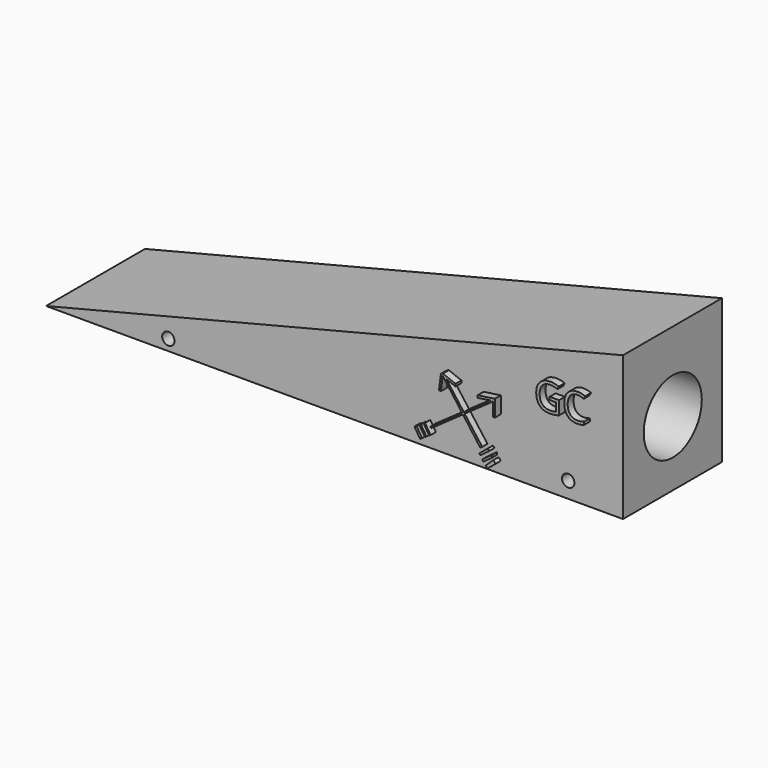
from build123d import *

# Parameters (mm, degrees)
F1_DEPTH     = 38.1
F4_DEPTH     = 2.032
F5_DEPTH     = 2.286
F6_R         = 11.180279411
F7_DEPTH     = 50.8
F8_TEXT_SIZE = 11.8700451114
F9_DEPTH     = 2.286
F11_DEPTH    = 3.302
F13_DEPTH    = 2.54
F14_R        = 1.905
F15_R        = 1.905
F16_DEPTH    = 58.166


# Not quite as in the source:
# - Text() gives the source's letters only with a copy of the font that has no kerning and outlines rounded to 1/6400 em; it was checked with that copy


with BuildPart() as f1:
    # F0 (on Front) → F1 (new body)
    with BuildSketch(Plane.XZ):
        Polygon((84.4861016917, 44.45), (-93.3138983083, 0), (84.4861016917, 0), align=None)
    extrude(amount=F1_DEPTH)

    # F2 (on face) → F4 (join)
    with BuildSketch(Plane.XZ.offset(38.1)):
        Polygon((36.5162249075, 14.0483667249), (26.7250510784, 7.1465180973), (26.9805269975, 6.7933419292), (36.7746398831, 13.6972623128), align=None)
        Polygon((30.2000753582, 22.6300209761), (36.5162249075, 14.0483667249), (37.0527973612, 14.4265993982), (30.6655891783, 22.9777331921), align=None)
        Polygon((37.0527973612, 14.4265993982), (36.5162249075, 14.0483667249), (36.7746398831, 13.6972623128), (37.3137278245, 14.0772681664), align=None)
        Polygon((46.3957208192, 21.0124740413), (37.0527973612, 14.4265993982), (37.3137278245, 14.0772681664), (46.6468408923, 20.6562274151), align=None)
        Polygon((37.3137278245, 14.0772681664), (36.7746398831, 13.6972623128), (42.1637693085, 6.3751358999), (42.7173138874, 6.8429983464), align=None)
        Polygon((26.8064830452, 4.8538930714), (25.0971019268, 7.6133394614), (24.6981563982, 7.2884358353), (26.3727214621, 4.5851928485), align=None)
        Polygon((23.8507352769, 6.7551592365), (23.2820510864, 6.3934870996), (25.0971019268, 3.7836717812), (25.5552400289, 4.0750387458), align=None)
        Polygon((22.5002579391, 5.9005115181), (21.8286830932, 5.5769649334), (23.5748943937, 2.7764131614), (24.2108590901, 3.1756572425), align=None)
        Polygon((44.4373336472, 6.9519355571), (41.8922938406, 4.8538930714), (42.146731168, 4.3679256923), (44.8550060391, 6.3934870996), align=None)
        Polygon((45.7004134124, 5.5769649334), (42.7396595478, 3.4473249689), (43.1043095887, 2.9500767123), (45.7004134124, 4.8538930714), align=None)
        Polygon((46.1449713403, 4.3679256923), (43.7690876424, 2.0963053685), (44.3023741245, 1.4547987375), (46.8240329698, 3.5510616751), align=None)
    extrude(amount=F4_DEPTH)

    # F3 (on face) → F5 (join)
    with BuildSketch(Plane.XZ.offset(38.1)):
        Polygon((30.8011006564, 22.9524802417), (30.2018001676, 22.6789433509), (29.5961014926, 18.046438694), (30.186894822, 17.9691926331), (30.7481582892, 22.2618479308), (34.7022227943, 20.7139663398), (34.7022227943, 21.4444510639), align=None)
        Polygon((46.8117631972, 21.3315784931), (41.5275767446, 20.5802936107), (41.5275767446, 19.8381505907), (46.1952015758, 20.5688290298), (46.1952015758, 16.2015352398), (46.8117631972, 16.2015352398), align=None)
    extrude(amount=F5_DEPTH)

    # F6 (on face) → F7 (cut)
    with BuildSketch(Plane.YZ.offset(84.4861016917)):
        with Locations((-18.9324077219, 20.0848150998)):
            Circle(F6_R)
    extrude(amount=-F7_DEPTH, mode=Mode.SUBTRACT)

    # F8 (on face) → F9 (join)
    with BuildSketch(Plane.XZ.offset(38.1)):
        with Locations((58.8393136859, 22.9422338307)):
            Text('GC', F8_TEXT_SIZE, font='Open Sans', text_align=(TextAlign.LEFT, TextAlign.BOTTOM))
    extrude(amount=F9_DEPTH)

    # F10 (on face) → F11 (join)
    with BuildSketch(Plane(origin=(0, 0, 0), x_dir=(-1, 0, 0), z_dir=(0, 1, 0))):
        with BuildLine():
            ThreePointArc((-60.3138038661, 23.5174087128), (-59.6757625272, 25.1334537281), (-59.4585558295, 26.8572633151))
            ThreePointArc((-59.4585558295, 26.8572633151), (-59.7265679953, 28.7685332219), (-60.5099305876, 30.5323717141))
            ThreePointArc((-60.5099305876, 30.5323717141), (-61.4176250088, 26.9967708953), (-60.3138038661, 23.5174087128))
        make_face()
        with BuildLine():
            ThreePointArc((-60.5099305876, 30.5323717141), (-59.7265679953, 28.7685332219), (-59.4585558295, 26.8572633151))
            ThreePointArc((-59.4585558295, 26.8572633151), (-59.6757625272, 25.1334537281), (-60.3138038661, 23.5174087128))
            ThreePointArc((-60.3138038661, 23.5174087128), (-60.0083497378, 23.0947919601), (-59.670587083, 22.697521859))
            Line((-59.670587083, 22.697521859), (-49.5405895639, 23.1574529709))
            ThreePointArc((-49.5405895639, 23.1574529709), (-48.5273645506, 25.0573141772), (-48.1772835424, 27.1818237249))
            ThreePointArc((-48.1772835424, 27.1818237249), (-53.06274754, 33.5716663476), (-60.5099305876, 30.5323717141))
        make_face()
        with BuildLine():
            ThreePointArc((-60.3138038661, 23.5174087128), (-61.4176250088, 26.9967708953), (-60.5099305876, 30.5323717141))
            ThreePointArc((-60.5099305876, 30.5323717141), (-70.6120653054, 32.3897694668), (-71.5275538512, 22.159181361))
            Line((-71.5275538512, 22.159181361), (-60.882702193, 22.6424883362))
            ThreePointArc((-60.882702193, 22.6424883362), (-60.5818049336, 23.0692535007), (-60.3138038661, 23.5174087128))
        make_face()
        with BuildLine():
            Line((-60.882702193, 22.6424883362), (-71.5275538512, 22.159181361))
            ThreePointArc((-71.5275538512, 22.159181361), (-66.0922869983, 19.9155076738), (-60.882702193, 22.6424883362))
        make_face()
        with BuildLine():
            ThreePointArc((-60.882702193, 22.6424883362), (-66.0922869983, 19.9155076738), (-71.5275538512, 22.159181361))
            Line((-71.5275538512, 22.159181361), (-59.9562898278, 9.5485188067))
            Line((-59.9562898278, 9.5485188067), (-49.5405895639, 23.1574529709))
            ThreePointArc((-49.5405895639, 23.1574529709), (-54.4984232888, 20.567174084), (-59.670587083, 22.697521859))
            Line((-59.670587083, 22.697521859), (-60.882702193, 22.6424883362))
        make_face()
        with BuildLine():
            Line((-49.5405895639, 23.1574529709), (-59.670587083, 22.697521859))
            ThreePointArc((-59.670587083, 22.697521859), (-54.4984232888, 20.567174084), (-49.5405895639, 23.1574529709))
        make_face()
    extrude(amount=F11_DEPTH)

    # F12 (on face) → F13 (join)
    with BuildSketch(Plane(origin=(0, 0, 0), x_dir=(-1, 0, 0), z_dir=(0, 1, 0))):
        Polygon((-45.9056382395, 29.9092462772), (-70.1136514434, 15.4644745257), (-68.9079016337, 14.443707731), (-45.0248309725, 28.7387271306), align=None)
        Polygon((-51.0166838108, 31.1331182486), (-45.9056382395, 29.9092462772), (-44.8613414473, 30.5323717141), (-44.1140569636, 29.283863571), (-45.0248309725, 28.7387271306), (-45.0248309725, 24.8769103405), (-43.3816564984, 24.8769103405), (-43.3816564984, 30.5323717141), (-51.1043375559, 32.6768323603), align=None)
        Polygon((-44.8613414473, 30.5323717141), (-45.9056382395, 29.9092462772), (-45.0248309725, 28.7387271306), (-44.1140569636, 29.283863571), align=None)
        Polygon((-73.425874103, 16.1324945134), (-74.4611546287, 15.4644745257), (-71.1798033989, 9.81955346), (-69.5808380732, 11.0227634054), align=None)
    extrude(amount=F13_DEPTH)

    # F14 (on face) + F15 (on face) → F16 (cut)
    with BuildSketch(Plane.XZ.offset(38.1)):
        with Locations((-55.632058531, 3.3839347307)):
            Circle(F14_R)
    with BuildSketch(Plane.XZ.offset(38.1)):
        with Locations((67.5919577479, 4.9378327094)):
            Circle(F15_R)
    extrude(amount=-F16_DEPTH, mode=Mode.SUBTRACT)


solid = f1.part
